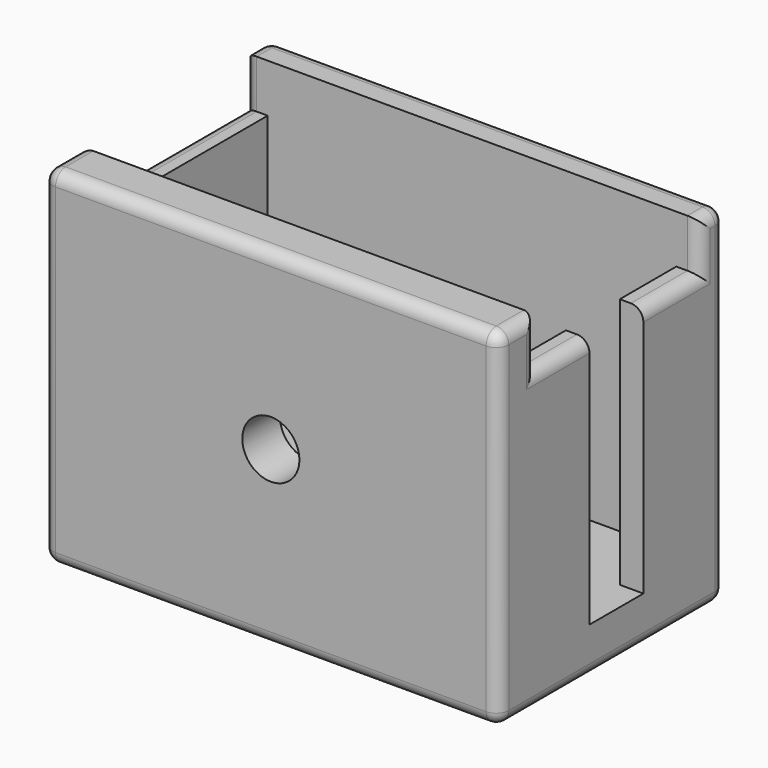
from build123d import *

# Parameters (mm, degrees)
F0_W     = 46.0375
F0_H     = 28.575
F1_DEPTH = 4.7625
F3_DEPTH = 30.2895
F2_W     = 2.38125
F2_H     = 20.6375
F4_DEPTH = 25.4
F6_DEPTH = 2.38125
F8_D     = 5.7658
F8_DEPTH = 4.7625
F8_TIP   = 1.7322210786
F9_R     = 1.27


# Not quite as in the source:
# - a feature names something its author has since deleted; it is built from what else it names


with BuildPart() as f1:
    # F0 (on Top) → F1 (new body)
    with BuildSketch(Plane.XY):
        Rectangle(F0_W, F0_H)
    extrude(amount=F1_DEPTH)

    # F2 (on face) → F3 (join)
    with BuildSketch(Plane.XY.offset(4.7625)):
        Polygon((-23.01875, -9.525), (-23.01875, -14.2875), (23.01875, -14.2875), (23.01875, -9.525), (20.6375, -9.525), (-20.6375, -9.525), align=None)
        Polygon((-23.01875, 14.2875), (-23.01875, 11.1125), (-20.6375, 11.1125), (20.6375, 11.1125), (23.01875, 11.1125), (23.01875, 14.2875), align=None)
    extrude(amount=F3_DEPTH)

    # F2 (on face) → F4 (join)
    with BuildSketch(Plane.XY.offset(4.7625)):
        Polygon((-23.01875, -9.525), (-23.01875, -14.2875), (23.01875, -14.2875), (23.01875, -9.525), (20.6375, -9.525), (-20.6375, -9.525), align=None)
        with Locations((-21.828125, 0.79375)):
            Rectangle(F2_W, F2_H)
        with Locations((21.828125, 0.79375)):
            Rectangle(F2_W, F2_H)
        Polygon((-23.01875, 14.2875), (-23.01875, 11.1125), (-20.6375, 11.1125), (20.6375, 11.1125), (23.01875, 11.1125), (23.01875, 14.2875), align=None)
    extrude(amount=F4_DEPTH)

    # F5 (on face) → F6 (cut, through all)
    with BuildSketch(Plane.YZ.offset(23.01875)):
        Polygon((3.9749178039, 30.1625), (0.3463463753, 30.1625), (-2.8286536247, 30.1625), (-2.8286536247, 16.5712326925), (-2.8286536247, 11.8087326925), (-2.8286536247, 4.7625), (0.3463463753, 4.7625), (3.9749178039, 4.7625), (3.9749178039, 16.5712326925), align=None)
    extrude(amount=-F6_DEPTH, mode=Mode.SUBTRACT)

    # F8
    with Locations(Plane.XZ.offset(14.2875)):
        with Locations((0, 17.526)):
            Hole(F8_D / 2, depth=F8_DEPTH)
            with Locations((0, 0, -(F8_DEPTH + F8_TIP / 2))):  # 118° drill point
                Cone(0, F8_D / 2, F8_TIP, mode=Mode.SUBTRACT)

    # F9
    f9_edges = [f1.edges().sort_by_distance(p)[0] for p in [
        (23.01875, 14.2875, 17.526),
        (-23.01875, 14.2875, 17.526),
        (0, 14.2875, 35.052),
        (0, 14.2875, 0),
        (23.01875, 0, 0),
        (-23.01875, 0, 0),
        (23.01875, 12.7, 35.052),
        (-23.01875, 12.7, 35.052),
        (23.01875, -14.2875, 17.526),
        (0, -14.2875, 35.052),
        (-23.01875, -14.2875, 17.526),
        (0, -14.2875, 0),
        (23.01875, -11.90625, 35.052),
        (-23.01875, -11.90625, 35.052),
        (-23.01875, 0.79375, 30.1625),
        (23.01875, 7.543709, 30.1625),
        (23.01875, -6.176827, 30.1625),
        (23.01875, -9.525, 32.60725),
        (-23.01875, -9.525, 32.60725),
        (-23.01875, 11.1125, 32.60725),
        (23.01875, 11.1125, 32.60725),
    ]]
    fillet(f9_edges, radius=F9_R)


solid = f1.part
